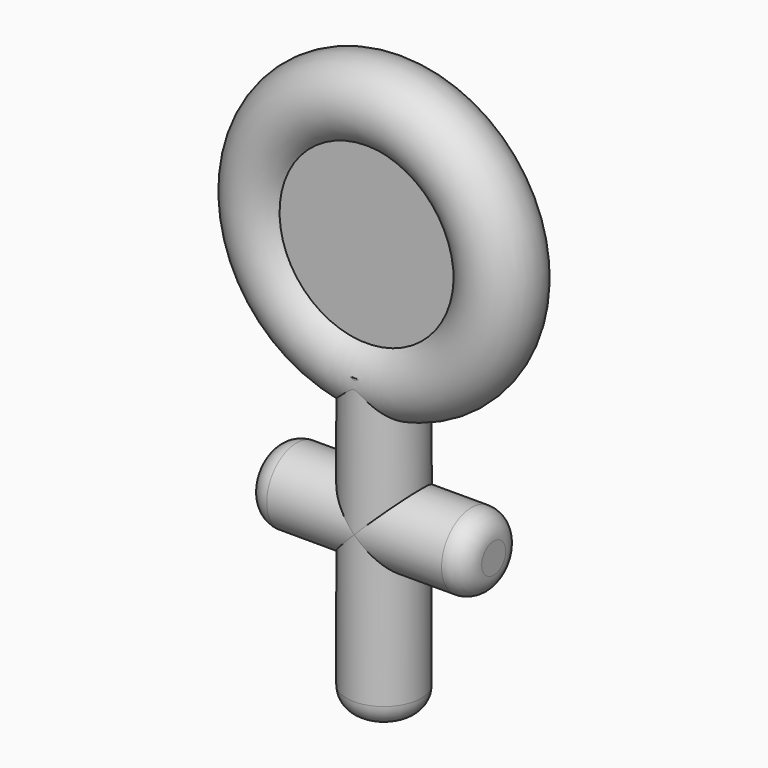
from build123d import *
from build123d import SkipClean  # not in build123d's __all__

# Parameters (mm, degrees)
F3_R     = 8.5
F4_DEPTH = 70
F5_R     = 5.08
F6_R     = 8.5
F7_DEPTH = 25
F8_R     = 5.08


# Not quite as in the source:
# - after a boolean that leaves OpenCascade's solid faulty, fix() repairs it


with BuildPart() as f1:
    # F0 (on Right) → F1 (revolve)
    with BuildSketch(Plane.YZ):
        with BuildLine():
            Line((4.9623605743, 0), (4.9623605743, 19.8352374136))
            ThreePointArc((4.9623605743, 19.8352374136), (0, 35.358186117), (-4.9623605743, 19.8352374136))
            Line((-4.9623605743, 19.8352374136), (-4.9623605743, 0))
            Line((-4.9623605743, 0), (0, 0))
            Line((0, 0), (4.9623605743, 0))
        make_face()
    revolve(axis=Axis((0, -2.4811802872, 0), (0, 1, 0)))

    # F3 (on offset) → F4 (join)
    with BuildSketch(Plane.XY.offset(-25.4)):
        Circle(F3_R)
    with SkipClean():  # cleaning this boolean's faces spoils the solid; the shape is the same uncleaned
        extrude(amount=-F4_DEPTH)

    # F5
    f5_edges = [f1.edges().sort_by_distance(p)[0] for p in [
        (-8.5, 0, -95.4),
    ]]
    fillet(f5_edges, radius=F5_R)

    # F6 (on Right) → F7 (join, symmetric)
    with BuildSketch(Plane.YZ):
        with Locations((0, -56.8226240575)):
            Circle(F6_R)
    extrude(amount=F7_DEPTH, both=True)

    add(f1.part.fix(), mode=Mode.REPLACE)

    # F8
    f8_edges = [f1.edges().sort_by_distance(p)[0] for p in [
        (-25, -8.5, -56.822624),
        (25, -8.5, -56.822624),
    ]]
    fillet(f8_edges, radius=F8_R)


solid = f1.part
